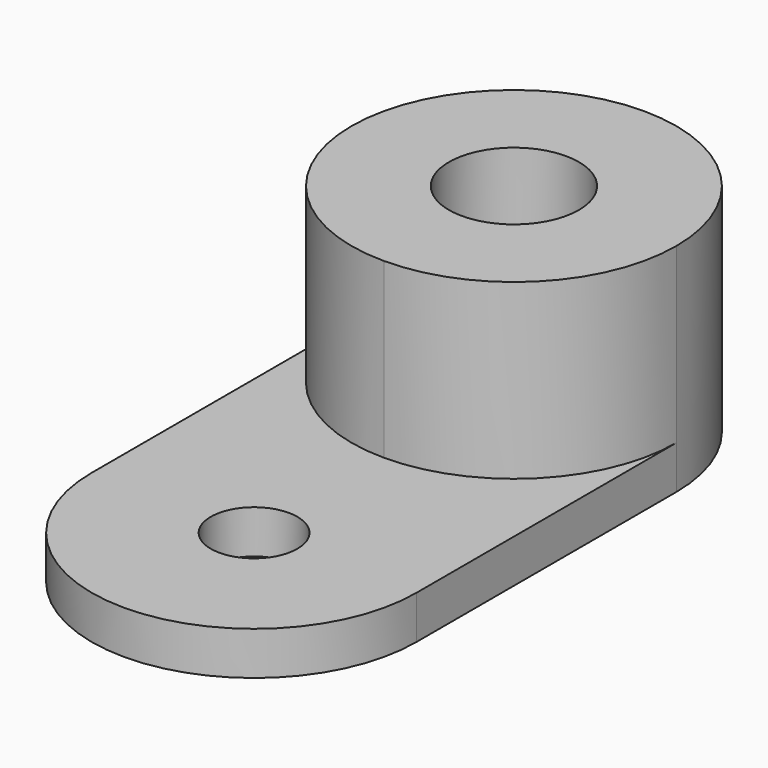
from build123d import *

# Parameters (mm, degrees)
F0_R     = 3
F1_DEPTH = 10
F0_R_2   = 2
F2_DEPTH = 2
F3_DEPTH = 5


# Not quite as in the source:
# - a feature names something its author has since deleted; it is built from what else it names


with BuildPart() as f1:
    # F0 (on Top) → F1 (new body)
    with BuildSketch(Plane.XY):
        with BuildLine():
            ThreePointArc((-7.5, 17.7205532079), (-5.303300866, 12.4172523561), (-2.02e-08, 10.2205532079))
            ThreePointArc((-2.02e-08, 10.2205532079), (5.3033008518, 12.4172523418), (7.5, 17.7205532079))
            ThreePointArc((7.5, 17.7205532079), (0, 25.2205532079), (-7.5, 17.7205532079))
        make_face()
        Polygon((-5.1134088242, 15.0398101151), (-4.8782960315, 20.8085236032), (0.2351127927, 23.489266696), (5.1134088242, 20.4012963006), (4.8782960315, 14.6325828125), (-0.2351127927, 11.9518397197), align=None, mode=Mode.SUBTRACT)
        Polygon((0.2351127927, 23.489266696), (-4.8782960315, 20.8085236032), (-5.1134088242, 15.0398101151), (-0.2351127927, 11.9518397197), (4.8782960315, 14.6325828125), (5.1134088242, 20.4012963006), align=None)
        with Locations((0, 17.7205532079)):
            Circle(F0_R, mode=Mode.SUBTRACT)
    extrude(amount=F1_DEPTH)

    # F0 (on Top) → F2 (join)
    with BuildSketch(Plane.XY):
        with BuildLine():
            ThreePointArc((-2.02e-08, 10.2205532079), (5.3033008518, 8.0238540739), (7.5, 2.7205532079))
            Line((7.5, 2.7205532079), (7.5, 17.7205532079))
            ThreePointArc((7.5, 17.7205532079), (5.3033008518, 12.4172523418), (-2.02e-08, 10.2205532079))
        make_face()
        with BuildLine():
            ThreePointArc((-2.02e-08, 10.2205532079), (-5.303300866, 8.0238540596), (-7.5, 2.7205532079))
            ThreePointArc((-7.5, 2.7205532079), (0, -4.7794467921), (7.5, 2.7205532079))
            ThreePointArc((7.5, 2.7205532079), (5.3033008518, 8.0238540739), (-2.02e-08, 10.2205532079))
        make_face()
        with Locations((0, 2.7205532079)):
            Circle(F0_R_2, mode=Mode.SUBTRACT)
        with BuildLine():
            Line((-7.5, 17.7205532079), (-7.5, 2.7205532079))
            ThreePointArc((-7.5, 2.7205532079), (-5.303300866, 8.0238540596), (-2.02e-08, 10.2205532079))
            ThreePointArc((-2.02e-08, 10.2205532079), (-5.303300866, 12.4172523561), (-7.5, 17.7205532079))
        make_face()
    extrude(amount=F2_DEPTH)

    # F0 (on Top) → F3 (cut)
    with BuildSketch(Plane.XY):
        Polygon((0.2351127927, 23.489266696), (-4.8782960315, 20.8085236032), (-5.1134088242, 15.0398101151), (-0.2351127927, 11.9518397197), (4.8782960315, 14.6325828125), (5.1134088242, 20.4012963006), align=None)
        with Locations((0, 17.7205532079)):
            Circle(F0_R, mode=Mode.SUBTRACT)
    extrude(amount=F3_DEPTH, mode=Mode.SUBTRACT)


solid = f1.part
